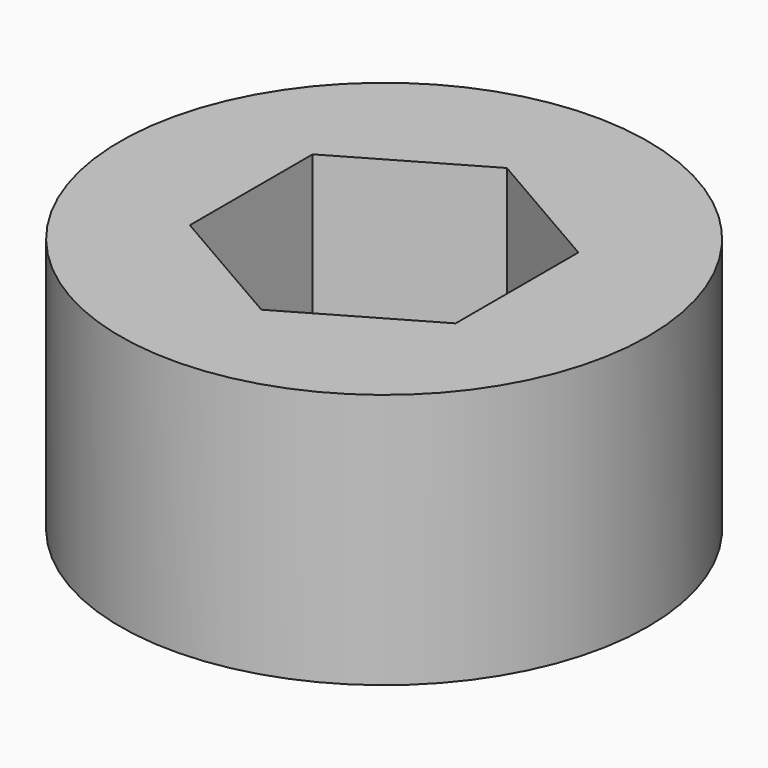
from build123d import *

# Parameters (mm, degrees)
F0_R     = 13.1191
F1_DEPTH = 12.7
F3_DEPTH = 36.322


# Not quite as in the source:
# - a length typed as a fraction of an inch, garbled in the dataset ("3 / 203.2 mm" for 3/8 in), is restored


with BuildPart() as f1:
    # F0 (on Top) → F1 (new body)
    with BuildSketch(Plane.XY):
        Circle(F0_R)
    extrude(amount=F1_DEPTH)

    # F2 (on Top) → F3 (cut)
    with BuildSketch(Plane.XY):
        Polygon((6.604, -3.8128211777), (6.604, 3.8128211777), (0, 7.6256423555), (-6.604, 3.8128211777), (-6.604, -3.8128211777), (0, -7.6256423555), align=None)
    extrude(amount=F3_DEPTH, mode=Mode.SUBTRACT)


solid = f1.part
